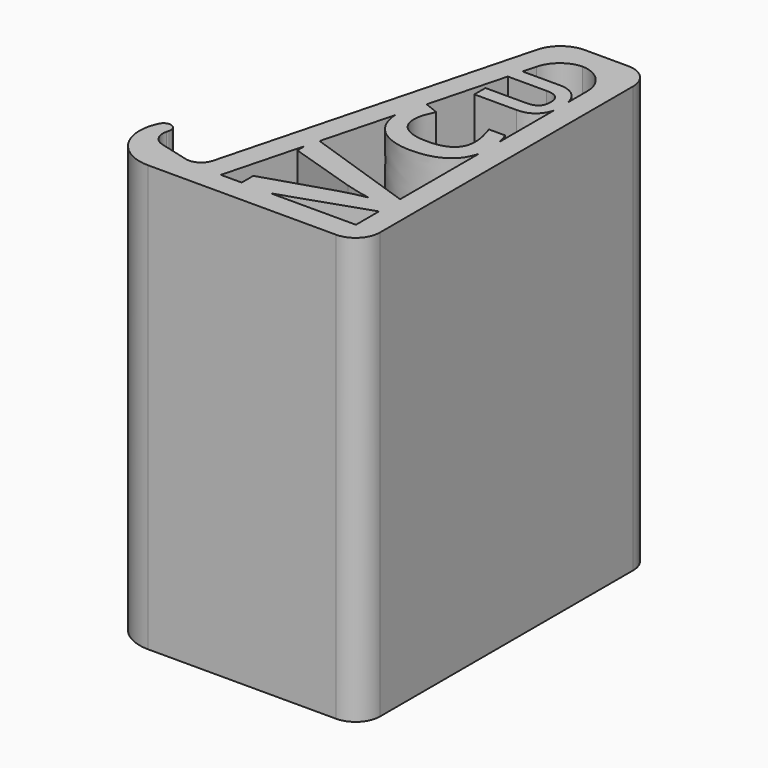
from build123d import *

# Parameters (mm, degrees)
F1_DEPTH       = 44.45
F2_R           = 3.175
F3_R           = 5.08
F4_R           = 6.35
F5_T1_DEPTH    = 88.9
F6_TEXT_SIZE   = 33.3854961387
F6_TEXT_SIZE_2 = 26.5476792297
F6_TEXT_SIZE_3 = 19.138222992
F7_DEPTH       = 44.45


# Not quite as in the source:
# - a fillet or chamfer that OpenCascade refuses, or shapes differently, is made with other operations: its cross-section is extruded or revolved along the edge and cut away or added
# - Text() gives the source's letters only with a copy of the font that has no kerning and outlines rounded to 1/6400 em; it was checked with that copy


with BuildPart() as f1:
    # F0 (on Top) → F1 (new body, symmetric)
    with BuildSketch(Plane.XY):
        with BuildLine():
            Line((-6.8987994573, -49.9839000404), (37.4415380651, -49.9839000404))
            Line((37.4415380651, -49.9839000404), (37.4415380651, 26.2160999596))
            Line((37.4415380651, 26.2160999596), (18.3915380651, 26.2160999596))
            Line((18.3915380651, 26.2160999596), (-0.4335921942, -45.2214000404))
            Line((-0.4335921942, -45.2214000404), (-12.7143470407, -41.9851892314))
            Line((-12.7143470407, -41.9851892314), (-11.7645760342, -38.3810034785))
            ThreePointArc((-11.7645760342, -38.3810034785), (-12.6876385857, -36.5716075939), (-14.5888685227, -37.2866479201))
            ThreePointArc((-14.5888685227, -37.2866479201), (-14.3210190316, -45.8017899925), (-6.8987994573, -49.9839000404))
        make_face()
        Polygon((4.4914918708, -45.2214000404), (22.0616134461, 21.4535999596), (32.6790380651, 21.4535999596), (32.6790380651, -45.2214000404), align=None, mode=Mode.SUBTRACT)
    extrude(amount=F1_DEPTH, both=True)

    # F2
    f2_edges = [f1.edges().sort_by_distance(p)[0] for p in [
        (-12.714347, -41.985189, 0),
        (-0.433592, -45.2214, 0),
    ]]
    fillet(f2_edges, radius=F2_R)

    # F3
    f3_edges = [f1.edges().sort_by_distance(p)[0] for p in [
        (37.441538, 26.2161, 0),
        (37.441538, -49.9839, 0),
    ]]
    fillet(f3_edges, radius=F3_R)

    # F4
    f4_edges = [f1.edges().sort_by_distance(p)[0] for p in [
        (18.391538, 26.2161, 0),
    ]]
    fillet(f4_edges, radius=F4_R)

    # F5: fillet of radius 6.35 on 2 edges, made by hand

    # F5_s2 → F5_t1 (join)
    with BuildSketch(Plane.XY.offset(-44.45)):
        with BuildLine():
            ThreePointArc((20.8146698642, 16.7217053641), (23.0789970632, 20.1333847124), (26.9550472874, 21.4535999596))
            Line((26.9550472874, 21.4535999596), (22.0616134461, 21.4535999596))
            Line((22.0616134461, 21.4535999596), (20.8146698642, 16.7217053641))
        make_face()
        with BuildLine():
            ThreePointArc((26.3290380651, 21.4535999596), (30.8191661256, 19.5937280201), (32.6790380651, 15.1035999596))
            Line((32.6790380651, 15.1035999596), (32.6790380651, 21.4535999596))
            Line((32.6790380651, 21.4535999596), (26.3290380651, 21.4535999596))
        make_face()
    extrude(amount=F5_T1_DEPTH)

    # F6 (on Top) → F7 (join, symmetric)
    with BuildSketch(Plane.XY):
        with Locations(Location((32.6790380651, -47.2876822337), (0, 0, 90))):
            Text('V', F6_TEXT_SIZE, font='Open Sans', font_style=FontStyle.BOLD, text_align=(TextAlign.LEFT, TextAlign.BOTTOM))
        with Locations(Location((32.6790380651, -20.6842157154), (0, 0, 90))):
            Text('C', F6_TEXT_SIZE_2, font='Open Sans', font_style=FontStyle.BOLD, text_align=(TextAlign.LEFT, TextAlign.BOTTOM))
        with Locations(Location((32.6790380651, 1.1257780228), (0, 0, 90))):
            Text('U', F6_TEXT_SIZE_3, font='Open Sans', font_style=FontStyle.BOLD, text_align=(TextAlign.LEFT, TextAlign.BOTTOM))
    extrude(amount=F7_DEPTH, both=True)


solid = f1.part
